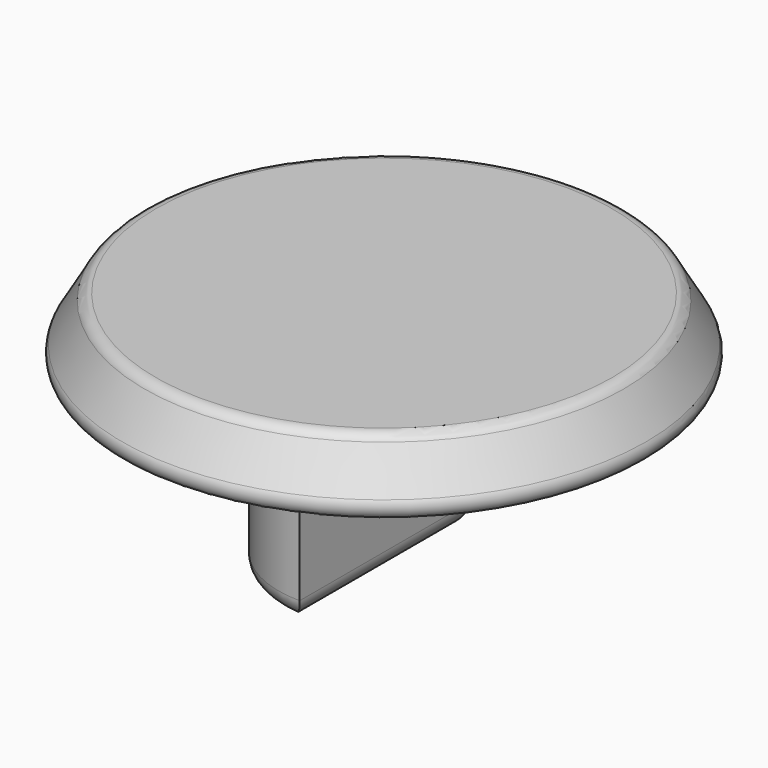
from build123d import *

# Parameters (mm, degrees)
F2_W     = 4.05
F2_H     = 8.1
F3_DEPTH = 6
F4_R     = 0.75
F5_R     = 0.5


with BuildPart() as f1:
    # F0 (on Front) → F1 (revolve)
    with BuildSketch(Plane.XZ):
        Polygon((4.05, 0), (4.05, 6), (5.5, 7), (10.5, 7), (9.056624327, 9.5), (0, 9.5), (0, 0), align=None)
    revolve(axis=Axis((0, 0, 4.75), (0, 0, -1)))

    # F2 (on face) → F3 (cut)
    with BuildSketch(Plane(origin=(0, 0, 0), x_dir=(1, 0, 0), z_dir=(0, 0, -1))):
        with Locations((2.025, 0)):
            Rectangle(F2_W, F2_H)
    extrude(amount=-F3_DEPTH, mode=Mode.SUBTRACT)

    # F4
    f4_edges = [f1.edges().sort_by_distance(p)[0] for p in [
        (0, 0, 0),
        (0, 0, 6),
        (-4.05, 0, 0),
    ]]
    fillet(f4_edges, radius=F4_R)

    # F5
    f5_edges = [f1.edges().sort_by_distance(p)[0] for p in [
        (-9.056624, 0, 9.5),
        (-10.5, 0, 7),
    ]]
    fillet(f5_edges, radius=F5_R)


solid = f1.part
